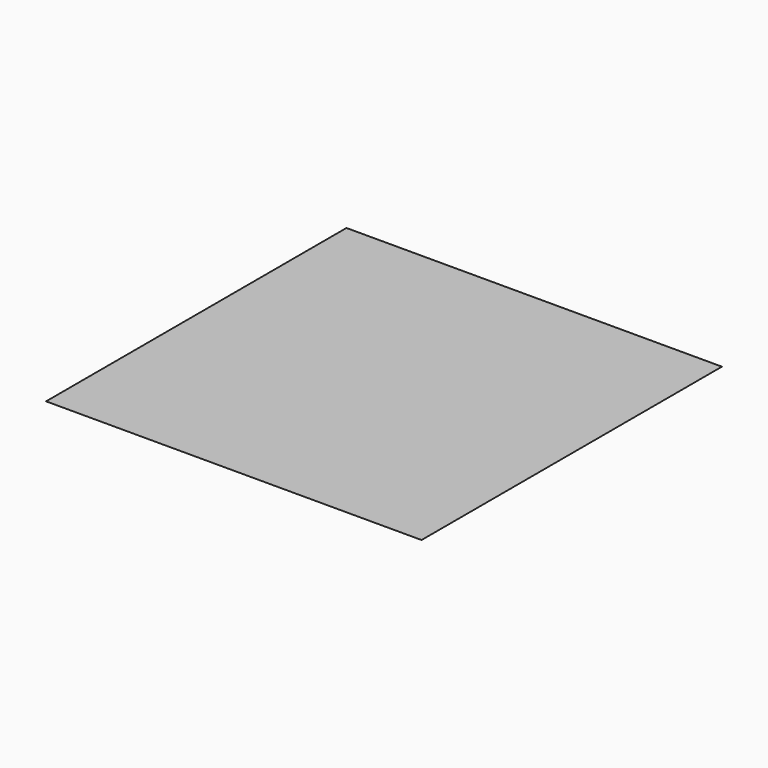
from build123d import *

# Parameters (mm, degrees)
F0_W     = 200
F0_H     = 200
F1_DEPTH = 10
F1_TAPER = 75


# Not quite as in the source:
# - a feature of the source that left no trace in its solid (it failed there, or was rolled back) is left out


with BuildPart() as f1:
    # F0 (on Top) → F1 (new body)
    with BuildSketch(Plane.XY):
        with Locations((-4.3254461373, -0.2492584803)):
            Rectangle(F0_W, F0_H)
    extrude(amount=-F1_DEPTH, taper=F1_TAPER)


solid = f1.part
